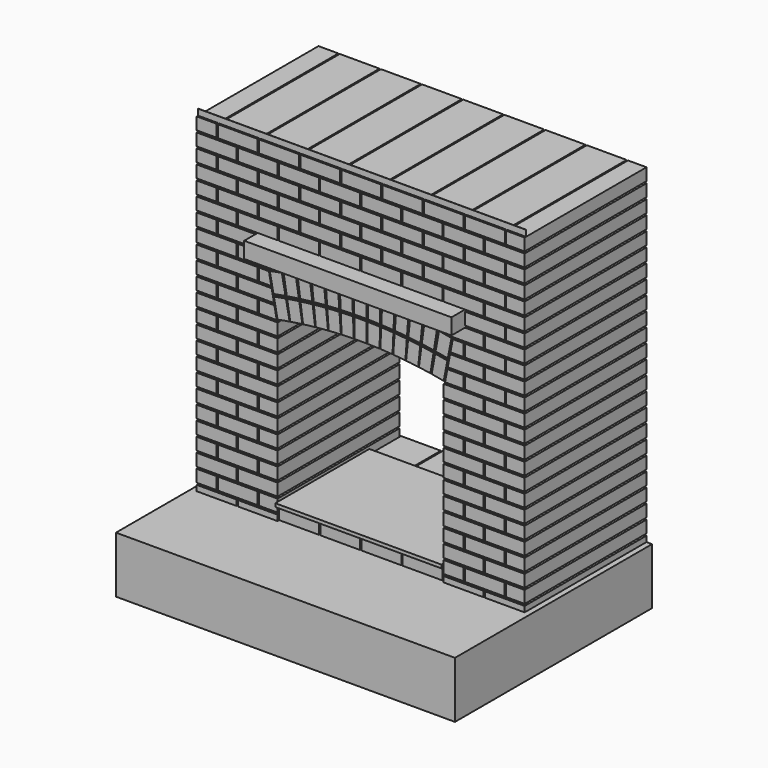
from build123d import *

# Parameters (mm, degrees)
F0_W          = 105.75
F0_H          = 65
F0_W_2        = 211.5
F0_W_3        = 98.25
F0_H_2        = 30
F0_W_4        = 105.25
F0_H_3        = 64.607629
F1_DEPTH      = 10
F1_DEPTH_BACK = 800
F2_DEPTH      = 25
F2_DEPTH_BACK = 600
F3_DEPTH      = 100
F4_DEPTH      = 510
F4_DEPTH_BACK = 800
F5_DEPTH      = 1


# Not quite as in the source:
# - ends of sketch curves that miss each other by under 0.0002 mm in the source are joined


with BuildPart() as f1:
    # F0 (on Front) → F1 (new body, two sides)
    with BuildSketch(Plane.XZ) as f1_sk:
        with Locations((-819.625, 978.6495302)):
            Rectangle(F0_W, F0_H)
        with Locations((-653.5, 978.6495302)):
            Rectangle(F0_W_2, F0_H)
        with Locations((-434.5, 978.6495302)):
            Rectangle(F0_W_2, F0_H)
        with Locations((-215.5, 978.6495302)):
            Rectangle(F0_W_2, F0_H)
        with Locations((3.5, 978.6495302)):
            Rectangle(F0_W_2, F0_H)
        with Locations((222.5, 978.6495302)):
            Rectangle(F0_W_2, F0_H)
        with Locations((441.5, 978.6495302)):
            Rectangle(F0_W_2, F0_H)
        with Locations((660.5, 978.6495302)):
            Rectangle(F0_W_2, F0_H)
        with Locations((822.875, 978.6495302)):
            Rectangle(F0_W_3, F0_H)
        with Locations((766.25, 903.6495302)):
            Rectangle(F0_W_2, F0_H)
        with Locations((-766.75, 903.6495302)):
            Rectangle(F0_W_2, F0_H)
        with Locations((-819.625, 828.6495302)):
            Rectangle(F0_W, F0_H)
        with Locations((-766.75, 753.6495302)):
            Rectangle(F0_W_2, F0_H)
        with Locations((-653.5, 828.6495302)):
            Rectangle(F0_W_2, F0_H)
        with Locations((-547.75, 903.6495302)):
            Rectangle(F0_W_2, F0_H)
        with Locations((-328.75, 903.6495302)):
            Rectangle(F0_W_2, F0_H)
        with Locations((-434.5, 828.6495302)):
            Rectangle(F0_W_2, F0_H)
        with Locations((-547.75, 753.6495302)):
            Rectangle(F0_W_2, F0_H)
        with Locations((-328.75, 753.6495302)):
            Rectangle(F0_W_2, F0_H)
        with Locations((-215.5, 828.6495302)):
            Rectangle(F0_W_2, F0_H)
        with Locations((-109.75, 903.6495302)):
            Rectangle(F0_W_2, F0_H)
        Polygon((-102.25, 861.1495302), (-102.25, 796.1495302), (109.25, 796.1495302), (109.25, 861.1495302), (3.5, 861.1495302), align=None)
        with Locations((-109.75, 753.6495302)):
            Rectangle(F0_W_2, F0_H)
        with Locations((109.25, 903.6495302)):
            Rectangle(F0_W_2, F0_H)
        Polygon((215, 861.1495302), (116.75, 861.1495302), (116.75, 796.1495302), (328.25, 796.1495302), (328.25, 861.1495302), align=None)
        with Locations((328.25, 903.6495302)):
            Rectangle(F0_W_2, F0_H)
        with Locations((441.5, 828.6495302)):
            Rectangle(F0_W_2, F0_H)
        with Locations((328.25, 753.6495302)):
            Rectangle(F0_W_2, F0_H)
        with Locations((547.25, 753.6495302)):
            Rectangle(F0_W_2, F0_H)
        with Locations((822.875, 828.6495302)):
            Rectangle(F0_W_3, F0_H)
        with Locations((766.25, 753.6495302)):
            Rectangle(F0_W_2, F0_H)
        with Locations((547.25, 903.6495302)):
            Rectangle(F0_W_2, F0_H)
        with Locations((660.5, 828.6495302)):
            Rectangle(F0_W_2, F0_H)
        with Locations((109.25, 753.6495302)):
            Rectangle(F0_W_2, F0_H)
        with Locations((-819.625, 678.6495302)):
            Rectangle(F0_W, F0_H)
        with Locations((-766.75, 603.6495302)):
            Rectangle(F0_W_2, F0_H)
        with Locations((-819.625, 528.6495302)):
            Rectangle(F0_W, F0_H)
        with Locations((-653.5, 528.6495302)):
            Rectangle(F0_W_2, F0_H)
        with Locations((-653.5, 678.6495302)):
            Rectangle(F0_W_2, F0_H)
        Polygon((-547.75, 571.1495302), (-442, 571.1495302), (-442, 636.1495302), (-653.5, 636.1495302), (-653.5, 571.1495302), align=None)
        with Locations((-434.5, 678.6495302)):
            Rectangle(F0_W_2, F0_H)
        with Locations((-328.75, 603.6495302)):
            Rectangle(F0_W_2, F0_H)
        with Locations((-215.5, 678.6495302)):
            Rectangle(F0_W_2, F0_H)
        with Locations((-109.75, 603.6495302)):
            Rectangle(F0_W_2, F0_H)
        with Locations((3.5, 678.6495302)):
            Rectangle(F0_W_2, F0_H)
        with Locations((109.25, 603.6495302)):
            Rectangle(F0_W_2, F0_H)
        with Locations((222.5, 678.6495302)):
            Rectangle(F0_W_2, F0_H)
        with Locations((328.25, 603.6495302)):
            Rectangle(F0_W_2, F0_H)
        with Locations((441.5, 678.6495302)):
            Rectangle(F0_W_2, F0_H)
        Polygon((441.5, 636.1495302), (441.5, 571.1495302), (554.75, 571.1495302), (653, 571.1495302), (653, 636.1495302), align=None)
        with Locations((660.5, 678.6495302)):
            Rectangle(F0_W_2, F0_H)
        with Locations((766.25, 603.6495302)):
            Rectangle(F0_W_2, F0_H)
        with Locations((822.875, 678.6495302)):
            Rectangle(F0_W_3, F0_H)
        with Locations((822.875, 528.6495302)):
            Rectangle(F0_W_3, F0_H)
        with Locations((660.5, 528.6495302)):
            Rectangle(F0_W_2, F0_H)
        with Locations((766.25, 453.6495302)):
            Rectangle(F0_W_2, F0_H)
        with BuildLine():
            Line((653, 486.1495302), (554.75, 486.1495302))
            Line((554.75, 486.1495302), (441.5, 486.1495302))
            Line((441.5, 486.1495302), (441.5, 429.1941382))
            ThreePointArc((441.5, 429.1941382), (463.318790633, 425.2664700416), (485.1026609901, 421.1495301488))
            Line((485.1026609901, 421.1495301488), (653, 421.1495302))
            Line((653, 421.1495302), (653, 486.1495302))
        make_face()
        with BuildLine():
            Line((434, 486.1495302), (222.5, 486.1495302))
            Line((222.5, 486.1495302), (222.5, 457.9377232))
            ThreePointArc((222.5, 457.9377232), (328.5365757301, 446.427387097), (434.0000000545, 430.4991305158))
            Line((434.0000000545, 430.4991305158), (434, 486.1495302))
        make_face()
        with BuildLine():
            Line((215, 486.1495302), (3.5, 486.1495302))
            Line((3.5, 486.1495302), (3.5, 467.6471312))
            ThreePointArc((3.5, 467.6471312), (109.3439714945, 465.3074471343), (215.0000000335, 458.582563596))
            Line((215.0000000335, 458.582563596), (215, 486.1495302))
        make_face()
        with BuildLine():
            Line((-4, 486.1495302), (-215.5, 486.1495302))
            Line((-215.5, 486.1495302), (-215.5, 458.5402672))
            ThreePointArc((-215.5, 458.5402672), (-109.8444031396, 465.2859502256), (-4.0000000003, 467.6463973929))
            Line((-4.0000000003, 467.6463973929), (-4, 486.1495302))
        make_face()
        with BuildLine():
            Line((-223, 486.1495302), (-434.5, 486.1495302))
            Line((-434.5, 486.1495302), (-434.5, 430.4128472))
            ThreePointArc((-434.5, 430.4128472), (-329.0370270242, 446.3624116177), (-223.0000000156, 457.8939413783))
            Line((-223.0000000156, 457.8939413783), (-223, 486.1495302))
        make_face()
        with BuildLine():
            Line((-442, 486.1495302), (-547.75, 486.1495302))
            Line((-547.75, 486.1495302), (-653.5, 486.1495302))
            Line((-653.5, 486.1495302), (-653.5, 421.1495302))
            Line((-653.5, 421.1495302), (-485.102661, 421.1495302))
            ThreePointArc((-485.1026609901, 421.1495301488), (-463.5684023211, 425.2204043328), (-442.0000000078, 429.1063192442))
            Line((-442, 429.1063192), (-442, 486.1495302))
        make_face()
        with Locations((-766.75, 453.6495302)):
            Rectangle(F0_W_2, F0_H)
        with Locations((-819.625, 378.6495302)):
            Rectangle(F0_W, F0_H)
        with Locations((-653.5, 378.6495302)):
            Rectangle(F0_W_2, F0_H)
        Polygon((-540.25, 346.1495302), (-475.3907933178, 346.1495302), (-487.9598097393, 411.1495302), (-540.25, 411.1495302), align=None)
        with Locations((-766.75, 303.6495302)):
            Rectangle(F0_W_2, F0_H)
        Polygon((-653.5, 271.1495302), (-460.8880820622, 271.1495302), (-473.4570984837, 336.1495302), (-653.5, 336.1495302), align=None)
        with Locations((-819.625, 228.6495302)):
            Rectangle(F0_W, F0_H)
        with Locations((-653.5, 228.6495302)):
            Rectangle(F0_W_2, F0_H)
        Polygon((-540.25, 196.1495302), (-446.3853708065, 196.1495302), (-446.909066112, 198.8577926219), (-458.9543872281, 261.1495302), (-540.25, 261.1495302), align=None)
        with Locations((-766.75, 153.6495302)):
            Rectangle(F0_W_2, F0_H)
        with Locations((-547.75, 153.6495302)):
            Rectangle(F0_W_2, F0_H)
        with Locations((-819.625, 78.6495302)):
            Rectangle(F0_W, F0_H)
        with Locations((-653.5, 78.6495302)):
            Rectangle(F0_W_2, F0_H)
        with Locations((-491.125, 78.6495302)):
            Rectangle(F0_W_3, F0_H)
        with Locations((-766.75, 3.6495302)):
            Rectangle(F0_W_2, F0_H)
        with Locations((-547.75, 3.6495302)):
            Rectangle(F0_W_2, F0_H)
        with Locations((-819.625, -71.3504698)):
            Rectangle(F0_W, F0_H)
        with Locations((-653.5, -71.3504698)):
            Rectangle(F0_W_2, F0_H)
        with Locations((-491.125, -71.3504698)):
            Rectangle(F0_W_3, F0_H)
        with Locations((-766.75, -146.3504698)):
            Rectangle(F0_W_2, F0_H)
        with Locations((-547.75, -146.3504698)):
            Rectangle(F0_W_2, F0_H)
        with Locations((-819.625, -221.3504698)):
            Rectangle(F0_W, F0_H)
        with Locations((-653.5, -221.3504698)):
            Rectangle(F0_W_2, F0_H)
        with Locations((-491.125, -221.3504698)):
            Rectangle(F0_W_3, F0_H)
        with Locations((-766.75, -296.3504698)):
            Rectangle(F0_W_2, F0_H)
        with Locations((-547.75, -296.3504698)):
            Rectangle(F0_W_2, F0_H)
        with Locations((-819.625, -371.3504698)):
            Rectangle(F0_W, F0_H)
        with Locations((-653.5, -371.3504698)):
            Rectangle(F0_W_2, F0_H)
        with Locations((-491.125, -371.3504698)):
            Rectangle(F0_W_3, F0_H)
        with Locations((-766.75, -446.3504698)):
            Rectangle(F0_W_2, F0_H)
        with Locations((-547.75, -446.3504698)):
            Rectangle(F0_W_2, F0_H)
        with Locations((-819.625, -521.3504698)):
            Rectangle(F0_W, F0_H)
        with Locations((-653.5, -521.3504698)):
            Rectangle(F0_W_2, F0_H)
        with Locations((-491.125, -521.3504698)):
            Rectangle(F0_W_3, F0_H)
        with Locations((-766.75, -596.3504698)):
            Rectangle(F0_W_2, F0_H)
        Polygon((-540.25, -628.8504698), (-442, -628.8504698), (-442, -563.8504698), (-540.25, -563.8504698), (-653.5, -563.8504698), (-653.5, -628.8504698), align=None)
        with Locations((-819.625, -671.3504698)):
            Rectangle(F0_W, F0_H)
        with Locations((-653.5, -671.3504698)):
            Rectangle(F0_W_2, F0_H)
        Polygon((-442, -671.8504698), (-442, -653.8504698), (-442, -638.8504698), (-540.25, -638.8504698), (-540.25, -703.8504698), (-442, -703.8504698), align=None)
        with Locations((-766.75, -728.8504698)):
            Rectangle(F0_W_2, F0_H_2)
        Polygon((-442, -743.8504698), (-442, -713.8504698), (-540.25, -713.8504698), (-653.5, -713.8504698), (-653.5, -743.8504698), align=None)
        with BuildLine():
            Line((-483.387866, 413.8422042), (-463.8330486219, 312.7155060601))
            ThreePointArc((-463.8330486219, 312.7155060601), (-431.8802658345, 318.6739780372), (-399.8510400321, 324.2068283936))
            Line((-399.8510400321, 324.2068283936), (-419.570047, 426.1826232))
            Line((-419.570047, 426.1826232), (-483.387866, 413.8422042))
        make_face()
        with BuildLine():
            ThreePointArc((-442.0000000511, 199.8070564643), (-410.0449024045, 205.7550928325), (-378.0098779423, 211.2564208495))
            Line((-378.0098779423, 211.2564208495), (-397.571998, 312.4208842))
            ThreePointArc((-397.571998, 312.4208842), (-429.6018040146, 306.891183884), (-461.5548179058, 300.933754713))
            Line((-461.5548179058, 300.933754713), (-442.0000000511, 199.8070564643))
        make_face()
        with BuildLine():
            Line((-345.255049, 436.6325702), (-409.542155, 426.9963582))
            Line((-409.542155, 426.9963582), (-392.97466, 325.3375522))
            ThreePointArc((-392.97466, 325.3375522), (-360.8602260561, 330.3522189595), (-328.6819200208, 334.9391973533))
            Line((-328.6819200208, 334.9391973533), (-345.255049, 436.6325702))
        make_face()
        with BuildLine():
            ThreePointArc((-374.4769660256, 211.8349733574), (-342.3605263553, 216.8391409049), (-310.1773530512, 221.3944395805))
            Line((-310.1773530512, 221.3944395805), (-326.751039, 323.0912352))
            ThreePointArc((-326.751039, 323.0912352), (-358.9298321954, 318.5074223666), (-391.044466044, 313.4938044698))
            Line((-391.044466044, 313.4938044698), (-374.4769660256, 211.8349733574))
        make_face()
        with BuildLine():
            ThreePointArc((-321.7752320422, 335.8668735179), (-289.5270191307, 339.933383771), (-257.2275600242, 343.5705094282))
            Line((-257.2275600242, 343.5705094282), (-270.797958, 445.7079412))
            Line((-270.797958, 445.7079412), (-335.341018, 437.9695962))
            Line((-335.341018, 437.9695962), (-321.7752320422, 335.8668735179))
        make_face()
        with BuildLine():
            ThreePointArc((-306.6289640133, 221.8686693005), (-274.3790547682, 225.9246255739), (-242.0756629788, 229.5299419976))
            Line((-242.0756629788, 229.5299419976), (-255.646518, 331.6708112))
            ThreePointArc((-255.646518, 331.6708112), (-287.9463704388, 328.0368642661), (-320.1947519369, 323.9714087251))
            Line((-320.1947519369, 323.9714087251), (-306.6289640133, 221.8686693005))
        make_face()
        with BuildLine():
            Line((-196.016445, 452.5930292), (-260.759648, 446.7615452))
            Line((-260.759648, 446.7615452), (-250.210954, 344.3031492))
            ThreePointArc((-250.210954, 344.3031492), (-217.8568398047, 347.4168338833), (-185.4641650184, 350.0998094411))
            Line((-185.4641650184, 350.0998094411), (-196.016445, 452.5930292))
        make_face()
        with BuildLine():
            ThreePointArc((-238.433284987, 229.9078410742), (-206.0777865672, 233.0109264045), (-173.6821190309, 235.661990613))
            Line((-173.6821190309, 235.661990613), (-184.234754, 338.1586602))
            ThreePointArc((-184.234754, 338.1586602), (-216.6277282892, 335.4788729431), (-248.9819800237, 332.3662474302))
            Line((-248.9819800237, 332.3662474302), (-238.433284987, 229.9078410742))
        make_face()
        with BuildLine():
            Line((-121.064406, 457.2696832), (-185.951429, 453.3501322))
            Line((-185.951429, 453.3501322), (-178.429004, 350.6251982))
            ThreePointArc((-178.429004, 350.6251982), (-145.9971352331, 352.7833488419), (-113.5394250016, 354.5098402354))
            Line((-113.5394250016, 354.5098402354), (-121.064406, 457.2696832))
        make_face()
        with BuildLine():
            ThreePointArc((-170.0301799999, 235.9323051992), (-137.5972403613, 238.0798200442), (-105.1374799791, 239.7743257379))
            Line((-105.1374799791, 239.7743257379), (-112.662714, 342.5376272))
            ThreePointArc((-112.662714, 342.5376272), (-145.120629789, 340.8143319749), (-177.5526050104, 338.6572443423))
            Line((-177.5526050104, 338.6572443423), (-170.0301799999, 235.9323051992))
        make_face()
        with BuildLine():
            Line((-46.007048, 459.7338352), (-110.981441, 457.7296252))
            Line((-110.981441, 457.7296252), (-106.49183, 354.8275212))
            ThreePointArc((-106.49183, 354.8275212), (-74.0104204152, 356.0282600205), (-41.5159110018, 356.7967653066))
            Line((-41.5159110018, 356.7967653066), (-46.007048, 459.7338352))
        make_face()
        with BuildLine():
            ThreePointArc((-75.0000000044, 240.9411613357), (-55.7525948236, 241.4818680956), (-36.5013759947, 241.8633698602))
            Line((-36.5013759947, 241.8633698602), (-40.992664, 344.8039042))
            ThreePointArc((-40.992664, 344.8039042), (-73.4872844958, 344.0385996794), (-105.9687690118, 342.8389264701))
            Line((-105.9687690118, 342.8389264701), (-101.479157, 239.9368202))
            ThreePointArc((-101.479157, 239.9368202), (-88.2410074228, 240.4766638217), (-75.0000000044, 240.9411613357))
        make_face()
        with BuildLine():
            Line((29.090335, 459.9833412), (-35.914904, 459.8962142))
            Line((-35.914904, 459.8962142), (-34.462013, 356.9064622))
            ThreePointArc((-34.4620130003, 356.9064622227), (-1.9593204, 357.1487445378), (30.5437189994, 356.9585951494))
            Line((30.543719, 356.9585952), (29.090335, 459.9833412))
        make_face()
        with BuildLine():
            ThreePointArc((-32.8398530067, 241.9179036746), (-0.3367183175, 242.1495058501), (32.1664820055, 241.9273055979))
            Line((32.1664820055, 241.9273055979), (30.713049, 344.9555192))
            ThreePointArc((30.713049, 344.9555192), (-1.7900074832, 345.1488712188), (-34.2927439988, 344.9076561152))
            Line((-34.2927439988, 344.9076561152), (-32.8398530067, 241.9179036746))
        make_face()
        with BuildLine():
            Line((104.16241, 458.0179842), (39.182878, 459.8480152))
            Line((39.182878, 459.8480152), (37.597785, 356.8602122))
            ThreePointArc((37.597785, 356.8602122), (70.0934852596, 356.143827617), (102.5767789897, 354.9951889544))
            Line((102.5767789897, 354.9951889544), (104.16241, 458.0179842))
        make_face()
        with BuildLine():
            ThreePointArc((75.0000000044, 240.9411613357), (87.9045305346, 240.4894018482), (100.8063570059, 239.9660773369))
            Line((100.8063570059, 239.9660773369), (102.392042, 342.9923402))
            ThreePointArc((102.392042, 342.9923402), (69.9088261653, 344.1441806532), (37.4131140046, 344.8616334979))
            Line((37.4131140046, 344.8616334979), (35.828021, 241.8738312))
            ThreePointArc((35.828021, 241.8738312), (55.4159726779, 241.4899072947), (75.0000000044, 240.9411613357))
        make_face()
        with BuildLine():
            Line((179.143869, 453.8394742), (114.246572, 457.5850682))
            Line((114.246572, 457.5850682), (109.624874, 354.6888122))
            ThreePointArc((109.624874, 354.6888122), (142.0853120166, 353.0143835036), (174.520600974, 350.9082548371))
            Line((174.520600974, 350.9082548371), (179.143869, 453.8394742))
        make_face()
        with BuildLine():
            ThreePointArc((104.4647260219, 239.8046406883), (136.9249753655, 238.1195244227), (169.3585350045, 235.981391262))
            Line((169.3585350045, 235.981391262), (173.981959, 338.9160752))
            ThreePointArc((173.981959, 338.9160752), (141.5468423868, 341.0254020347), (109.0864240213, 342.7008986747))
            Line((109.0864240213, 342.7008986747), (104.4647260219, 239.8046406883))
        make_face()
        with BuildLine():
            Line((253.969481, 447.4514462), (189.210877, 453.1093432))
            Line((189.210877, 453.1093432), (181.556595, 350.3941502))
            ThreePointArc((181.556595, 350.3941502), (213.9535313724, 347.763134652), (246.3125980045, 344.7013482448))
            Line((246.3125980045, 344.7013482448), (253.969481, 447.4514462))
        make_face()
        with BuildLine():
            ThreePointArc((173.0105519895, 235.7121330592), (205.4069846582, 233.0704398176), (237.7633789655, 229.976713864))
            Line((237.7633789655, 229.976713864), (245.42052, 332.7302702))
            ThreePointArc((245.42052, 332.7302702), (213.0617195995, 335.7952485431), (180.6648340136, 338.427331383))
            Line((180.6648340136, 338.427331383), (173.0105519895, 235.7121330592))
        make_face()
        with BuildLine():
            Line((328.574151, 438.8594582), (264.010577, 446.4247342))
            Line((264.010577, 446.4247342), (253.33037, 343.9799632))
            ThreePointArc((253.33037, 343.9799632), (285.6356212129, 340.3946494003), (317.8903149526, 336.3798688386))
            Line((317.8903149526, 336.3798688386), (328.574151, 438.8594582))
        make_face()
        with BuildLine():
            Line((305.961381, 221.9572692), (316.645576, 324.4403072))
            ThreePointArc((316.645576, 324.4403072), (284.3912427335, 328.4582702099), (252.0860740238, 332.0446494287))
            Line((252.0860740238, 332.0446494287), (241.405867, 229.5998682))
            ThreePointArc((241.405867, 229.5998682), (273.7103000729, 226.0038961985), (305.961381, 221.9572692))
        make_face()
        with BuildLine():
            Line((405.599474, 427.6357542), (338.580599, 437.5370562))
            Line((338.580599, 437.5370562), (324.88376, 335.4518312))
            ThreePointArc((324.88376, 335.4518312), (357.0692220657, 330.9153378912), (389.1914829385, 325.9510558191))
            Line((389.1914829385, 325.9510558191), (405.599474, 427.6357542))
        make_face()
        with BuildLine():
            Line((323.288012, 323.5584052), (309.59117, 221.4731632))
            ThreePointArc((309.59117, 221.4731632), (340.2616386282, 217.1502064186), (370.8718809386, 212.4195968195))
            Line((370.8718809386, 212.4195968195), (387.279872, 314.1042952))
            ThreePointArc((387.279872, 314.1042952), (355.3153873438, 319.044193727), (323.288012, 323.5584052))
        make_face()
        with BuildLine():
            ThreePointArc((398.2221910504, 324.4764905053), (430.8047181498, 318.8669007094), (463.3083509699, 312.8169070443))
            Line((463.3083509699, 312.8169070443), (482.841047, 413.9478802))
            Line((482.841047, 413.9478802), (416.775209, 425.8069112))
            Line((416.775209, 425.8069112), (398.2221910504, 324.4764905053))
        make_face()
        with BuildLine():
            Line((396.060659, 312.6709242), (377.507375, 211.3390512))
            ThreePointArc((377.507375, 211.3390512), (409.5436020977, 205.8447308744), (441.5000000537, 199.9036844779))
            Line((441.5000000537, 199.9036844779), (461.0326965703, 301.0346578085))
            ThreePointArc((461.0326965703, 301.0346578085), (428.5861708433, 307.0733027072), (396.060659, 312.6709242))
        make_face()
        Polygon((477.384909, 346.1495302), (547.25, 346.1495302), (547.25, 411.1495302), (489.939176, 411.1495302), align=None)
        with Locations((660.5, 378.6495302)):
            Rectangle(F0_W_2, F0_H)
        with Locations((822.875, 378.6495302)):
            Rectangle(F0_W_3, F0_H)
        Polygon((462.899216, 271.1495302), (653, 271.1495302), (653, 336.1495302), (475.453483, 336.1495302), align=None)
        with Locations((766.25, 303.6495302)):
            Rectangle(F0_W_2, F0_H)
        Polygon((448.413522, 196.1495302), (547.25, 196.1495302), (547.25, 261.1495302), (460.96779, 261.1495302), align=None)
        with Locations((660.5, 228.6495302)):
            Rectangle(F0_W_2, F0_H)
        with Locations((822.875, 228.6495302)):
            Rectangle(F0_W_3, F0_H)
        with Locations((547.25, 153.6495302)):
            Rectangle(F0_W_2, F0_H)
        with Locations((766.25, 153.6495302)):
            Rectangle(F0_W_2, F0_H)
        with Locations((494.125, 78.6495302)):
            Rectangle(F0_W_4, F0_H)
        Polygon((554.25, 46.1495302), (765.75, 46.1495302), (765.75, 111.1495302), (660.5, 111.1495302), (554.25, 111.1495302), align=None)
        Polygon((871.5, 46.1495302), (872, 46.1495302), (872, 111.1495302), (773.25, 111.1495302), (773.25, 46.1495302), align=None)
        with Locations((547.25, 3.6495302)):
            Rectangle(F0_W_2, F0_H)
        with Locations((766.25, 3.6495302)):
            Rectangle(F0_W_2, F0_H)
        with Locations((494.125, -71.3504698)):
            Rectangle(F0_W_4, F0_H)
        Polygon((554.25, -103.8504698), (765.75, -103.8504698), (765.75, -38.8504698), (660.5, -38.8504698), (554.25, -38.8504698), align=None)
        Polygon((871.5, -103.8504698), (872, -103.8504698), (872, -38.8504698), (773.25, -38.8504698), (773.25, -103.8504698), align=None)
        with Locations((547.25, -146.3504698)):
            Rectangle(F0_W_2, F0_H)
        with Locations((766.25, -146.3504698)):
            Rectangle(F0_W_2, F0_H)
        with Locations((494.125, -221.3504698)):
            Rectangle(F0_W_4, F0_H)
        Polygon((554.25, -253.8504698), (765.75, -253.8504698), (765.75, -188.8504698), (660.5, -188.8504698), (554.25, -188.8504698), align=None)
        Polygon((871.5, -253.8504698), (872, -253.8504698), (872, -188.8504698), (773.25, -188.8504698), (773.25, -253.8504698), align=None)
        with Locations((547.25, -296.3504698)):
            Rectangle(F0_W_2, F0_H)
        with Locations((766.25, -296.3504698)):
            Rectangle(F0_W_2, F0_H)
        with Locations((494.125, -371.3504698)):
            Rectangle(F0_W_4, F0_H)
        Polygon((554.25, -403.8504698), (765.75, -403.8504698), (765.75, -338.8504698), (660.5, -338.8504698), (554.25, -338.8504698), align=None)
        Polygon((871.5, -403.8504698), (872, -403.8504698), (872, -338.8504698), (773.25, -338.8504698), (773.25, -403.8504698), align=None)
        with Locations((547.25, -446.3504698)):
            Rectangle(F0_W_2, F0_H)
        with Locations((766.25, -446.3504698)):
            Rectangle(F0_W_2, F0_H)
        with Locations((494.125, -521.3504698)):
            Rectangle(F0_W_4, F0_H)
        Polygon((554.25, -553.8504698), (765.75, -553.8504698), (765.75, -488.8504698), (660.5, -488.8504698), (554.25, -488.8504698), align=None)
        Polygon((871.5, -553.8504698), (872, -553.8504698), (872, -488.8504698), (773.25, -488.8504698), (773.25, -553.8504698), align=None)
        with Locations((547.25, -596.3504698)):
            Rectangle(F0_W_2, F0_H)
        with Locations((766.25, -596.3504698)):
            Rectangle(F0_W_2, F0_H)
        Polygon((546.75, -638.8504698), (441.5, -638.8504698), (441.5, -653.8504698), (441.5, -671.8504698), (441.5, -703.8504698), (546.75, -703.8504698), align=None)
        Polygon((554.25, -703.8504698), (765.75, -703.8504698), (765.75, -638.8504698), (660.5, -638.8504698), (554.25, -638.8504698), align=None)
        Polygon((871.5, -703.8504698), (872, -703.8504698), (872, -638.8504698), (773.25, -638.8504698), (773.25, -703.8504698), align=None)
        with Locations((547.25, -728.8504698)):
            Rectangle(F0_W_2, F0_H_2)
        with Locations((766.25, -728.8504698)):
            Rectangle(F0_W_2, F0_H_2)
        with Locations((-327.566109, -704.1542843)):
            Rectangle(F0_W_2, F0_H_3)
        Polygon((-2.816109, -671.8504698), (-214.316109, -671.8504698), (-214.316109, -736.4580988), (-101.066109, -736.4580988), (-2.816109, -736.4580988), align=None)
        with Locations((110.433891, -704.1542843)):
            Rectangle(F0_W_2, F0_H_3)
        with Locations((329.433891, -704.1542843)):
            Rectangle(F0_W_2, F0_H_3)
    extrude(amount=F1_DEPTH)
    extrude(f1_sk.sketch, amount=-F1_DEPTH_BACK)


with BuildPart() as f2:
    # F0 (on Front) → F2 (new body, two sides)
    with BuildSketch(Plane.XZ) as f2_sk:
        Polygon((441.5, -671.8504698), (441.5, -653.8504698), (-442, -653.8504698), (-442, -671.8504698), (-433.316109, -671.8504698), (-221.816109, -671.8504698), (-214.316109, -671.8504698), (-2.816109, -671.8504698), (4.683891, -671.8504698), (216.183891, -671.8504698), (223.683891, -671.8504698), (435.183891, -671.8504698), align=None)
    extrude(amount=F2_DEPTH)
    extrude(f2_sk.sketch, amount=-F2_DEPTH_BACK)


with BuildPart() as f3:
    # F0 (on Front) → F3 (new body)
    with BuildSketch(Plane.XZ):
        Polygon((-434.5, 571.1495302), (-442, 571.1495302), (-547.75, 571.1495302), (-547.75, 561.1495302), (-547.75, 496.1495302), (-547.75, 486.1495302), (-442, 486.1495302), (-434.5, 486.1495302), (-223, 486.1495302), (-215.5, 486.1495302), (-4, 486.1495302), (3.5, 486.1495302), (215, 486.1495302), (222.5, 486.1495302), (434, 486.1495302), (441.5, 486.1495302), (554.75, 486.1495302), (554.75, 496.1495302), (554.75, 561.1495302), (554.75, 571.1495302), (441.5, 571.1495302), (434, 571.1495302), (222.5, 571.1495302), (215, 571.1495302), (3.5, 571.1495302), (-4, 571.1495302), (-215.5, 571.1495302), (-223, 571.1495302), align=None)
    extrude(amount=F3_DEPTH)


with BuildPart() as f4:
    # F0 (on Front) → F4 (new body, two sides)
    with BuildSketch(Plane.XZ) as f4_sk:
        Polygon((653, -743.8504698), (441.5, -743.8504698), (2.5, -743.8504698), (-95.75, -743.8504698), (-103.25, -743.8504698), (-314.75, -743.8504698), (-322.25, -743.8504698), (-428, -743.8504698), (-442, -743.8504698), (-653.5, -743.8504698), (-661, -743.8504698), (-872.5, -743.8504698), (-901.5, -743.8504698), (-901.5, -1043.8504698), (901.5, -1043.8504698), (901.5, -743.8504698), (872, -743.8504698), (660.5, -743.8504698), align=None)
    extrude(amount=F4_DEPTH)
    extrude(f4_sk.sketch, amount=-F4_DEPTH_BACK)


with BuildPart() as f5:
    # F0 (on Front) → F5 (new body)
    with BuildSketch(Plane.XZ):
        with BuildLine():
            ThreePointArc((252.0860740238, 332.0446494287), (284.3912427335, 328.4582702099), (316.6455760142, 324.4403073079))
            Line((316.6455760142, 324.4403073079), (305.961381, 221.9572692))
            ThreePointArc((305.961381, 221.9572692), (307.7763706985, 221.7159299891), (309.5911700875, 221.4731638524))
            Line((309.5911700875, 221.4731638524), (323.288012, 323.5584052))
            ThreePointArc((323.288012, 323.5584052), (355.3153873438, 319.044193727), (387.2798719572, 314.1042949345))
            Line((387.2798719572, 314.1042949345), (370.871881, 212.4195972))
            ThreePointArc((370.871881, 212.4195972), (374.190018025, 211.8817192921), (377.5073750406, 211.3390514471))
            Line((377.5073750406, 211.3390514471), (396.060659, 312.6709242))
            ThreePointArc((396.060659, 312.6709242), (428.5861708433, 307.0733027072), (461.0326969117, 301.0346577426))
            Line((461.0326969117, 301.0346577426), (441.5, 199.9036842))
            Line((441.5, 199.9036842), (441.5, 186.1495302))
            Line((441.5, 186.1495302), (653, 186.1495302))
            Line((653, 186.1495302), (653, 121.1495302))
            Line((653, 121.1495302), (441.5, 121.1495302))
            Line((441.5, 121.1495302), (441.5, 111.1495302))
            Line((441.5, 111.1495302), (546.75, 111.1495302))
            Line((546.75, 111.1495302), (546.75, 46.1495302))
            Line((546.75, 46.1495302), (441.5, 46.1495302))
            Line((441.5, 46.1495302), (441.5, 36.1495302))
            Line((441.5, 36.1495302), (653, 36.1495302))
            Line((653, 36.1495302), (653, -28.8504698))
            Line((653, -28.8504698), (441.5, -28.8504698))
            Line((441.5, -28.8504698), (441.5, -38.8504698))
            Line((441.5, -38.8504698), (546.75, -38.8504698))
            Line((546.75, -38.8504698), (546.75, -103.8504698))
            Line((546.75, -103.8504698), (441.5, -103.8504698))
            Line((441.5, -103.8504698), (441.5, -113.8504698))
            Line((441.5, -113.8504698), (653, -113.8504698))
            Line((653, -113.8504698), (653, -178.8504698))
            Line((653, -178.8504698), (441.5, -178.8504698))
            Line((441.5, -178.8504698), (441.5, -188.8504698))
            Line((441.5, -188.8504698), (546.75, -188.8504698))
            Line((546.75, -188.8504698), (546.75, -253.8504698))
            Line((546.75, -253.8504698), (441.5, -253.8504698))
            Line((441.5, -253.8504698), (441.5, -263.8504698))
            Line((441.5, -263.8504698), (653, -263.8504698))
            Line((653, -263.8504698), (653, -328.8504698))
            Line((653, -328.8504698), (441.5, -328.8504698))
            Line((441.5, -328.8504698), (441.5, -338.8504698))
            Line((441.5, -338.8504698), (546.75, -338.8504698))
            Line((546.75, -338.8504698), (546.75, -403.8504698))
            Line((546.75, -403.8504698), (441.5, -403.8504698))
            Line((441.5, -403.8504698), (441.5, -413.8504698))
            Line((441.5, -413.8504698), (653, -413.8504698))
            Line((653, -413.8504698), (653, -478.8504698))
            Line((653, -478.8504698), (441.5, -478.8504698))
            Line((441.5, -478.8504698), (441.5, -488.8504698))
            Line((441.5, -488.8504698), (546.75, -488.8504698))
            Line((546.75, -488.8504698), (546.75, -553.8504698))
            Line((546.75, -553.8504698), (441.5, -553.8504698))
            Line((441.5, -553.8504698), (441.5, -563.8504698))
            Line((441.5, -563.8504698), (653, -563.8504698))
            Line((653, -563.8504698), (653, -628.8504698))
            Line((653, -628.8504698), (441.5, -628.8504698))
            Line((441.5, -628.8504698), (441.5, -638.8504698))
            Line((441.5, -638.8504698), (546.75, -638.8504698))
            Line((546.75, -638.8504698), (546.75, -703.8504698))
            Line((546.75, -703.8504698), (441.5, -703.8504698))
            Line((441.5, -703.8504698), (441.5, -713.8504698))
            Line((441.5, -713.8504698), (653, -713.8504698))
            Line((653, -713.8504698), (653, -743.8504698))
            Line((653, -743.8504698), (660.5, -743.8504698))
            Line((660.5, -743.8504698), (660.5, -713.8504698))
            Line((660.5, -713.8504698), (872, -713.8504698))
            Line((872, -713.8504698), (872, -703.8504698))
            Line((872, -703.8504698), (871.5, -703.8504698))
            Line((871.5, -703.8504698), (773.25, -703.8504698))
            Line((773.25, -703.8504698), (773.25, -638.8504698))
            Line((773.25, -638.8504698), (872, -638.8504698))
            Line((872, -638.8504698), (872, -628.8504698))
            Line((872, -628.8504698), (660.5, -628.8504698))
            Line((660.5, -628.8504698), (660.5, -563.8504698))
            Line((660.5, -563.8504698), (872, -563.8504698))
            Line((872, -563.8504698), (872, -553.8504698))
            Line((872, -553.8504698), (871.5, -553.8504698))
            Line((871.5, -553.8504698), (773.25, -553.8504698))
            Line((773.25, -553.8504698), (773.25, -488.8504698))
            Line((773.25, -488.8504698), (872, -488.8504698))
            Line((872, -488.8504698), (872, -478.8504698))
            Line((872, -478.8504698), (660.5, -478.8504698))
            Line((660.5, -478.8504698), (660.5, -413.8504698))
            Line((660.5, -413.8504698), (872, -413.8504698))
            Line((872, -413.8504698), (872, -403.8504698))
            Line((872, -403.8504698), (871.5, -403.8504698))
            Line((871.5, -403.8504698), (773.25, -403.8504698))
            Line((773.25, -403.8504698), (773.25, -338.8504698))
            Line((773.25, -338.8504698), (872, -338.8504698))
            Line((872, -338.8504698), (872, -328.8504698))
            Line((872, -328.8504698), (660.5, -328.8504698))
            Line((660.5, -328.8504698), (660.5, -263.8504698))
            Line((660.5, -263.8504698), (872, -263.8504698))
            Line((872, -263.8504698), (872, -253.8504698))
            Line((872, -253.8504698), (871.5, -253.8504698))
            Line((871.5, -253.8504698), (773.25, -253.8504698))
            Line((773.25, -253.8504698), (773.25, -188.8504698))
            Line((773.25, -188.8504698), (872, -188.8504698))
            Line((872, -188.8504698), (872, -178.8504698))
            Line((872, -178.8504698), (660.5, -178.8504698))
            Line((660.5, -178.8504698), (660.5, -113.8504698))
            Line((660.5, -113.8504698), (872, -113.8504698))
            Line((872, -113.8504698), (872, -103.8504698))
            Line((872, -103.8504698), (871.5, -103.8504698))
            Line((871.5, -103.8504698), (773.25, -103.8504698))
            Line((773.25, -103.8504698), (773.25, -38.8504698))
            Line((773.25, -38.8504698), (872, -38.8504698))
            Line((872, -38.8504698), (872, -28.8504698))
            Line((872, -28.8504698), (660.5, -28.8504698))
            Line((660.5, -28.8504698), (660.5, 36.1495302))
            Line((660.5, 36.1495302), (872, 36.1495302))
            Line((872, 36.1495302), (872, 46.1495302))
            Line((872, 46.1495302), (871.5, 46.1495302))
            Line((871.5, 46.1495302), (773.25, 46.1495302))
            Line((773.25, 46.1495302), (773.25, 111.1495302))
            Line((773.25, 111.1495302), (872, 111.1495302))
            Line((872, 111.1495302), (872, 121.1495302))
            Line((872, 121.1495302), (660.5, 121.1495302))
            Line((660.5, 121.1495302), (660.5, 186.1495302))
            Line((660.5, 186.1495302), (872, 186.1495302))
            Line((872, 186.1495302), (872, 196.1495302))
            Line((872, 196.1495302), (773.75, 196.1495302))
            Line((773.75, 196.1495302), (773.75, 261.1495302))
            Line((773.75, 261.1495302), (872, 261.1495302))
            Line((872, 261.1495302), (872, 271.1495302))
            Line((872, 271.1495302), (660.5, 271.1495302))
            Line((660.5, 271.1495302), (660.5, 336.1495302))
            Line((660.5, 336.1495302), (872, 336.1495302))
            Line((872, 336.1495302), (872, 346.1495302))
            Line((872, 346.1495302), (773.75, 346.1495302))
            Line((773.75, 346.1495302), (773.75, 411.1495302))
            Line((773.75, 411.1495302), (872, 411.1495302))
            Line((872, 411.1495302), (872, 421.1495302))
            Line((872, 421.1495302), (660.5, 421.1495302))
            Line((660.5, 421.1495302), (660.5, 486.1495302))
            Line((660.5, 486.1495302), (872, 486.1495302))
            Line((872, 486.1495302), (872, 496.1495302))
            Line((872, 496.1495302), (773.75, 496.1495302))
            Line((773.75, 496.1495302), (773.75, 561.1495302))
            Line((773.75, 561.1495302), (872, 561.1495302))
            Line((872, 561.1495302), (872, 571.1495302))
            Line((872, 571.1495302), (660.5, 571.1495302))
            Line((660.5, 571.1495302), (660.5, 636.1495302))
            Line((660.5, 636.1495302), (872, 636.1495302))
            Line((872, 636.1495302), (872, 646.1495302))
            Line((872, 646.1495302), (773.75, 646.1495302))
            Line((773.75, 646.1495302), (773.75, 711.1495302))
            Line((773.75, 711.1495302), (872, 711.1495302))
            Line((872, 711.1495302), (872, 721.1495302))
            Line((872, 721.1495302), (660.5, 721.1495302))
            Line((660.5, 721.1495302), (660.5, 786.1495302))
            Line((660.5, 786.1495302), (872, 786.1495302))
            Line((872, 786.1495302), (872, 796.1495302))
            Line((872, 796.1495302), (773.75, 796.1495302))
            Line((773.75, 796.1495302), (773.75, 861.1495302))
            Line((773.75, 861.1495302), (872, 861.1495302))
            Line((872, 861.1495302), (872, 871.1495302))
            Line((872, 871.1495302), (660.5, 871.1495302))
            Line((660.5, 871.1495302), (660.5, 936.1495302))
            Line((660.5, 936.1495302), (872, 936.1495302))
            Line((872, 936.1495302), (872, 946.1495302))
            Line((872, 946.1495302), (773.75, 946.1495302))
            Line((773.75, 946.1495302), (773.75, 1011.1495302))
            Line((773.75, 1011.1495302), (872, 1011.1495302))
            Line((872, 1011.1495302), (872, 1043.8504952))
            Line((872, 1043.8504952), (-872.5, 1043.8504952))
            Line((-872.5, 1043.8504952), (-872.5, 1011.1495302))
            Line((-872.5, 1011.1495302), (-766.75, 1011.1495302))
            Line((-766.75, 1011.1495302), (-766.75, 946.1495302))
            Line((-766.75, 946.1495302), (-872.5, 946.1495302))
            Line((-872.5, 946.1495302), (-872.5, 936.1495302))
            Line((-872.5, 936.1495302), (-661, 936.1495302))
            Line((-661, 936.1495302), (-661, 871.1495302))
            Line((-661, 871.1495302), (-872.5, 871.1495302))
            Line((-872.5, 871.1495302), (-872.5, 861.1495302))
            Line((-872.5, 861.1495302), (-766.75, 861.1495302))
            Line((-766.75, 861.1495302), (-766.75, 796.1495302))
            Line((-766.75, 796.1495302), (-872.5, 796.1495302))
            Line((-872.5, 796.1495302), (-872.5, 786.1495302))
            Line((-872.5, 786.1495302), (-661, 786.1495302))
            Line((-661, 786.1495302), (-661, 721.1495302))
            Line((-661, 721.1495302), (-872.5, 721.1495302))
            Line((-872.5, 721.1495302), (-872.5, 711.1495302))
            Line((-872.5, 711.1495302), (-766.75, 711.1495302))
            Line((-766.75, 711.1495302), (-766.75, 646.1495302))
            Line((-766.75, 646.1495302), (-872.5, 646.1495302))
            Line((-872.5, 646.1495302), (-872.5, 636.1495302))
            Line((-872.5, 636.1495302), (-661, 636.1495302))
            Line((-661, 636.1495302), (-661, 571.1495302))
            Line((-661, 571.1495302), (-872.5, 571.1495302))
            Line((-872.5, 571.1495302), (-872.5, 561.1495302))
            Line((-872.5, 561.1495302), (-766.75, 561.1495302))
            Line((-766.75, 561.1495302), (-766.75, 496.1495302))
            Line((-766.75, 496.1495302), (-872.5, 496.1495302))
            Line((-872.5, 496.1495302), (-872.5, 486.1495302))
            Line((-872.5, 486.1495302), (-661, 486.1495302))
            Line((-661, 486.1495302), (-661, 421.1495302))
            Line((-661, 421.1495302), (-872.5, 421.1495302))
            Line((-872.5, 421.1495302), (-872.5, 411.1495302))
            Line((-872.5, 411.1495302), (-766.75, 411.1495302))
            Line((-766.75, 411.1495302), (-766.75, 346.1495302))
            Line((-766.75, 346.1495302), (-872.5, 346.1495302))
            Line((-872.5, 346.1495302), (-872.5, 336.1495302))
            Line((-872.5, 336.1495302), (-661, 336.1495302))
            Line((-661, 336.1495302), (-661, 271.1495302))
            Line((-661, 271.1495302), (-872.5, 271.1495302))
            Line((-872.5, 271.1495302), (-872.5, 261.1495302))
            Line((-872.5, 261.1495302), (-766.75, 261.1495302))
            Line((-766.75, 261.1495302), (-766.75, 196.1495302))
            Line((-766.75, 196.1495302), (-872.5, 196.1495302))
            Line((-872.5, 196.1495302), (-872.5, 186.1495302))
            Line((-872.5, 186.1495302), (-661, 186.1495302))
            Line((-661, 186.1495302), (-661, 121.1495302))
            Line((-661, 121.1495302), (-872.5, 121.1495302))
            Line((-872.5, 121.1495302), (-872.5, 111.1495302))
            Line((-872.5, 111.1495302), (-766.75, 111.1495302))
            Line((-766.75, 111.1495302), (-766.75, 46.1495302))
            Line((-766.75, 46.1495302), (-872.5, 46.1495302))
            Line((-872.5, 46.1495302), (-872.5, 36.1495302))
            Line((-872.5, 36.1495302), (-661, 36.1495302))
            Line((-661, 36.1495302), (-661, -28.8504698))
            Line((-661, -28.8504698), (-872.5, -28.8504698))
            Line((-872.5, -28.8504698), (-872.5, -38.8504698))
            Line((-872.5, -38.8504698), (-766.75, -38.8504698))
            Line((-766.75, -38.8504698), (-766.75, -103.8504698))
            Line((-766.75, -103.8504698), (-872.5, -103.8504698))
            Line((-872.5, -103.8504698), (-872.5, -113.8504698))
            Line((-872.5, -113.8504698), (-661, -113.8504698))
            Line((-661, -113.8504698), (-661, -178.8504698))
            Line((-661, -178.8504698), (-872.5, -178.8504698))
            Line((-872.5, -178.8504698), (-872.5, -188.8504698))
            Line((-872.5, -188.8504698), (-766.75, -188.8504698))
            Line((-766.75, -188.8504698), (-766.75, -253.8504698))
            Line((-766.75, -253.8504698), (-872.5, -253.8504698))
            Line((-872.5, -253.8504698), (-872.5, -263.8504698))
            Line((-872.5, -263.8504698), (-661, -263.8504698))
            Line((-661, -263.8504698), (-661, -328.8504698))
            Line((-661, -328.8504698), (-872.5, -328.8504698))
            Line((-872.5, -328.8504698), (-872.5, -338.8504698))
            Line((-872.5, -338.8504698), (-766.75, -338.8504698))
            Line((-766.75, -338.8504698), (-766.75, -403.8504698))
            Line((-766.75, -403.8504698), (-872.5, -403.8504698))
            Line((-872.5, -403.8504698), (-872.5, -413.8504698))
            Line((-872.5, -413.8504698), (-661, -413.8504698))
            Line((-661, -413.8504698), (-661, -478.8504698))
            Line((-661, -478.8504698), (-872.5, -478.8504698))
            Line((-872.5, -478.8504698), (-872.5, -488.8504698))
            Line((-872.5, -488.8504698), (-766.75, -488.8504698))
            Line((-766.75, -488.8504698), (-766.75, -553.8504698))
            Line((-766.75, -553.8504698), (-872.5, -553.8504698))
            Line((-872.5, -553.8504698), (-872.5, -563.8504698))
            Line((-872.5, -563.8504698), (-661, -563.8504698))
            Line((-661, -563.8504698), (-661, -628.8504698))
            Line((-661, -628.8504698), (-872.5, -628.8504698))
            Line((-872.5, -628.8504698), (-872.5, -638.8504698))
            Line((-872.5, -638.8504698), (-766.75, -638.8504698))
            Line((-766.75, -638.8504698), (-766.75, -703.8504698))
            Line((-766.75, -703.8504698), (-872.5, -703.8504698))
            Line((-872.5, -703.8504698), (-872.5, -713.8504698))
            Line((-872.5, -713.8504698), (-661, -713.8504698))
            Line((-661, -713.8504698), (-661, -743.8504698))
            Line((-661, -743.8504698), (-653.5, -743.8504698))
            Line((-653.5, -743.8504698), (-653.5, -713.8504698))
            Line((-653.5, -713.8504698), (-540.25, -713.8504698))
            Line((-540.25, -713.8504698), (-442, -713.8504698))
            Line((-442, -713.8504698), (-442, -703.8504698))
            Line((-442, -703.8504698), (-540.25, -703.8504698))
            Line((-540.25, -703.8504698), (-540.25, -638.8504698))
            Line((-540.25, -638.8504698), (-442, -638.8504698))
            Line((-442, -638.8504698), (-442, -628.8504698))
            Line((-442, -628.8504698), (-540.25, -628.8504698))
            Line((-540.25, -628.8504698), (-653.5, -628.8504698))
            Line((-653.5, -628.8504698), (-653.5, -563.8504698))
            Line((-653.5, -563.8504698), (-540.25, -563.8504698))
            Line((-540.25, -563.8504698), (-442, -563.8504698))
            Line((-442, -563.8504698), (-442, -553.8504698))
            Line((-442, -553.8504698), (-540.25, -553.8504698))
            Line((-540.25, -553.8504698), (-540.25, -488.8504698))
            Line((-540.25, -488.8504698), (-442, -488.8504698))
            Line((-442, -488.8504698), (-442, -478.8504698))
            Line((-442, -478.8504698), (-653.5, -478.8504698))
            Line((-653.5, -478.8504698), (-653.5, -413.8504698))
            Line((-653.5, -413.8504698), (-442, -413.8504698))
            Line((-442, -413.8504698), (-442, -403.8504698))
            Line((-442, -403.8504698), (-540.25, -403.8504698))
            Line((-540.25, -403.8504698), (-540.25, -338.8504698))
            Line((-540.25, -338.8504698), (-442, -338.8504698))
            Line((-442, -338.8504698), (-442, -328.8504698))
            Line((-442, -328.8504698), (-653.5, -328.8504698))
            Line((-653.5, -328.8504698), (-653.5, -263.8504698))
            Line((-653.5, -263.8504698), (-442, -263.8504698))
            Line((-442, -263.8504698), (-442, -253.8504698))
            Line((-442, -253.8504698), (-540.25, -253.8504698))
            Line((-540.25, -253.8504698), (-540.25, -188.8504698))
            Line((-540.25, -188.8504698), (-442, -188.8504698))
            Line((-442, -188.8504698), (-442, -178.8504698))
            Line((-442, -178.8504698), (-653.5, -178.8504698))
            Line((-653.5, -178.8504698), (-653.5, -113.8504698))
            Line((-653.5, -113.8504698), (-442, -113.8504698))
            Line((-442, -113.8504698), (-442, -103.8504698))
            Line((-442, -103.8504698), (-540.25, -103.8504698))
            Line((-540.25, -103.8504698), (-540.25, -38.8504698))
            Line((-540.25, -38.8504698), (-442, -38.8504698))
            Line((-442, -38.8504698), (-442, -28.8504698))
            Line((-442, -28.8504698), (-653.5, -28.8504698))
            Line((-653.5, -28.8504698), (-653.5, 36.1495302))
            Line((-653.5, 36.1495302), (-442, 36.1495302))
            Line((-442, 36.1495302), (-442, 46.1495302))
            Line((-442, 46.1495302), (-540.25, 46.1495302))
            Line((-540.25, 46.1495302), (-540.25, 111.1495302))
            Line((-540.25, 111.1495302), (-442, 111.1495302))
            Line((-442, 111.1495302), (-442, 121.1495302))
            Line((-442, 121.1495302), (-653.5, 121.1495302))
            Line((-653.5, 121.1495302), (-653.5, 186.1495302))
            Line((-653.5, 186.1495302), (-442, 186.1495302))
            Line((-442, 186.1495302), (-442, 199.8070562))
            Line((-442, 199.8070562), (-461.5548174667, 300.9337547979))
            ThreePointArc((-461.5548174667, 300.9337547979), (-429.6018040146, 306.891183884), (-397.5719980529, 312.4208845189))
            Line((-397.5719980529, 312.4208845189), (-378.009878, 211.2564212))
            ThreePointArc((-378.009878, 211.2564212), (-376.2435331896, 211.5463761767), (-374.4769660256, 211.8349733574))
            Line((-374.4769660256, 211.8349733574), (-391.044466, 313.4938042))
            ThreePointArc((-391.044466, 313.4938042), (-358.9298321954, 318.5074223666), (-326.7510390134, 323.0912352991))
            Line((-326.7510390134, 323.0912352991), (-310.177353, 221.3944392))
            ThreePointArc((-310.177353, 221.3944392), (-308.4032496848, 221.6322364825), (-306.6289640133, 221.8686693005))
            Line((-306.6289640133, 221.8686693005), (-320.194752, 323.9714092))
            ThreePointArc((-320.194752, 323.9714092), (-287.9463704388, 328.0368642661), (-255.6465180267, 331.6708114522))
            Line((-255.6465180267, 331.6708114522), (-242.075663, 229.5299422))
            ThreePointArc((-242.075663, 229.5299422), (-240.2545482832, 229.7196076782), (-238.433284987, 229.9078410742))
            Line((-238.433284987, 229.9078410742), (-248.98198, 332.3662472))
            ThreePointArc((-248.98198, 332.3662472), (-216.6277282892, 335.4788729431), (-184.2347539717, 338.1586598273))
            Line((-184.2347539717, 338.1586598273), (-173.682119, 235.6619902))
            ThreePointArc((-173.682119, 235.6619902), (-171.856202663, 235.7978659283), (-170.0301799999, 235.9323051992))
            Line((-170.0301799999, 235.9323051992), (-177.552605, 338.6572442))
            ThreePointArc((-177.552605, 338.6572442), (-145.120629789, 340.8143319749), (-112.6627140026, 342.5376272557))
            Line((-112.6627140026, 342.5376272557), (-105.13748, 239.7743262))
            ThreePointArc((-105.13748, 239.7743262), (-103.3083504479, 239.8562924667), (-101.4791570192, 239.9368206406))
            Line((-101.4791570192, 239.9368206406), (-105.968769, 342.8389262))
            ThreePointArc((-105.968769, 342.8389262), (-73.4872844958, 344.0385996794), (-40.9926639998, 344.8039041901))
            Line((-40.9926639998, 344.8039041901), (-36.501376, 241.8633702))
            ThreePointArc((-36.501376, 241.8633702), (-34.6706252228, 241.8913566738), (-32.8398530067, 241.9179036746))
            Line((-32.8398530067, 241.9179036746), (-34.292744, 344.9076562))
            ThreePointArc((-34.292744, 344.9076562), (-1.7900074832, 345.1488712188), (30.7130489994, 344.9555191553))
            Line((30.7130489994, 344.9555191553), (32.166482, 241.9273052))
            ThreePointArc((32.166482, 241.9273052), (33.9972620145, 241.9012881678), (35.8280209957, 241.8738309184))
            Line((35.8280209957, 241.8738309184), (37.413114, 344.8616332))
            ThreePointArc((37.413114, 344.8616332), (69.9088261653, 344.1441806532), (102.3920420016, 342.9923402389))
            Line((102.3920420016, 342.9923402389), (100.806357, 239.9660772))
            ThreePointArc((100.806357, 239.9660772), (102.6355732546, 239.8860782989), (104.4647260219, 239.8046406883))
            Line((104.4647260219, 239.8046406883), (109.086424, 342.7008982))
            ThreePointArc((109.086424, 342.7008982), (141.5468423868, 341.0254020347), (173.981959008, 338.9160753115))
            Line((173.981959008, 338.9160753115), (169.358535, 235.9813912))
            ThreePointArc((169.358535, 235.9813912), (171.1845964369, 235.8474801981), (173.0105519895, 235.7121330592))
            Line((173.0105519895, 235.7121330592), (180.664834, 338.4273312))
            ThreePointArc((180.664834, 338.4273312), (213.0617195995, 335.7952485431), (245.4205200321, 332.7302705164))
            Line((245.4205200321, 332.7302705164), (237.763379, 229.9767142))
            ThreePointArc((237.763379, 229.9767142), (239.5846970817, 229.7890072518), (241.4058670116, 229.5998683114))
            Line((241.4058670116, 229.5998683114), (252.0860740238, 332.0446494287))
        make_face()
        with Locations((-653.5, -671.3504698)):
            Rectangle(F0_W_2, F0_H, mode=Mode.SUBTRACT)
        with Locations((-653.5, -521.3504698)):
            Rectangle(F0_W_2, F0_H, mode=Mode.SUBTRACT)
        with Locations((-653.5, -371.3504698)):
            Rectangle(F0_W_2, F0_H, mode=Mode.SUBTRACT)
        with Locations((-653.5, -221.3504698)):
            Rectangle(F0_W_2, F0_H, mode=Mode.SUBTRACT)
        with Locations((-653.5, -71.3504698)):
            Rectangle(F0_W_2, F0_H, mode=Mode.SUBTRACT)
        Polygon((765.75, -638.8504698), (765.75, -703.8504698), (554.25, -703.8504698), (554.25, -638.8504698), (660.5, -638.8504698), align=None, mode=Mode.SUBTRACT)
        Polygon((765.75, -488.8504698), (765.75, -553.8504698), (554.25, -553.8504698), (554.25, -488.8504698), (660.5, -488.8504698), align=None, mode=Mode.SUBTRACT)
        Polygon((765.75, -338.8504698), (765.75, -403.8504698), (554.25, -403.8504698), (554.25, -338.8504698), (660.5, -338.8504698), align=None, mode=Mode.SUBTRACT)
        Polygon((765.75, -188.8504698), (765.75, -253.8504698), (554.25, -253.8504698), (554.25, -188.8504698), (660.5, -188.8504698), align=None, mode=Mode.SUBTRACT)
        Polygon((765.75, -38.8504698), (765.75, -103.8504698), (554.25, -103.8504698), (554.25, -38.8504698), (660.5, -38.8504698), align=None, mode=Mode.SUBTRACT)
        with Locations((-653.5, 78.6495302)):
            Rectangle(F0_W_2, F0_H, mode=Mode.SUBTRACT)
        with Locations((-653.5, 228.6495302)):
            Rectangle(F0_W_2, F0_H, mode=Mode.SUBTRACT)
        Polygon((-446.909066112, 198.8577926219), (-446.3853708065, 196.1495302), (-540.25, 196.1495302), (-540.25, 261.1495302), (-458.9543872281, 261.1495302), align=None, mode=Mode.SUBTRACT)
        with Locations((-653.5, 378.6495302)):
            Rectangle(F0_W_2, F0_H, mode=Mode.SUBTRACT)
        Polygon((-473.4570984837, 336.1495302), (-460.8880820622, 271.1495302), (-653.5, 271.1495302), (-653.5, 336.1495302), align=None, mode=Mode.SUBTRACT)
        Polygon((-487.9598097393, 411.1495302), (-475.3907933178, 346.1495302), (-540.25, 346.1495302), (-540.25, 411.1495302), align=None, mode=Mode.SUBTRACT)
        with BuildLine():
            ThreePointArc((-399.8510400321, 324.2068283936), (-431.8802658345, 318.6739780372), (-463.8330489603, 312.7155059946))
            Line((-463.8330489603, 312.7155059946), (-483.387866, 413.8422042))
            Line((-483.387866, 413.8422042), (-419.570047, 426.1826232))
            Line((-419.570047, 426.1826232), (-399.8510400321, 324.2068283936))
        make_face(mode=Mode.SUBTRACT)
        with BuildLine():
            Line((-392.97466, 325.3375522), (-409.542155, 426.9963582))
            Line((-409.542155, 426.9963582), (-345.255049, 436.6325702))
            Line((-345.255049, 436.6325702), (-328.68192, 334.9391972))
            ThreePointArc((-328.68192, 334.9391972), (-360.8602260561, 330.3522189595), (-392.97466, 325.3375522))
        make_face(mode=Mode.SUBTRACT)
        with BuildLine():
            Line((-270.797958, 445.7079412), (-257.22756, 343.5705092))
            ThreePointArc((-257.22756, 343.5705092), (-289.5270191307, 339.933383771), (-321.7752320422, 335.8668735179))
            Line((-321.7752320422, 335.8668735179), (-335.341018, 437.9695962))
            Line((-335.341018, 437.9695962), (-270.797958, 445.7079412))
        make_face(mode=Mode.SUBTRACT)
        with BuildLine():
            Line((-250.210954, 344.3031492), (-260.759648, 446.7615452))
            Line((-260.759648, 446.7615452), (-196.016445, 452.5930292))
            Line((-196.016445, 452.5930292), (-185.464165, 350.0998092))
            ThreePointArc((-185.464165, 350.0998092), (-217.8568398047, 347.4168338833), (-250.210954, 344.3031492))
        make_face(mode=Mode.SUBTRACT)
        with BuildLine():
            Line((-178.429004, 350.6251982), (-185.951429, 453.3501322))
            Line((-185.951429, 453.3501322), (-121.064406, 457.2696832))
            Line((-121.064406, 457.2696832), (-113.539425, 354.5098402))
            ThreePointArc((-113.539425, 354.5098402), (-145.9971352331, 352.7833488419), (-178.429004, 350.6251982))
        make_face(mode=Mode.SUBTRACT)
        with BuildLine():
            Line((-106.49183, 354.8275212), (-110.981441, 457.7296252))
            Line((-110.981441, 457.7296252), (-46.007048, 459.7338352))
            Line((-46.007048, 459.7338352), (-41.515911, 356.7967652))
            ThreePointArc((-41.515911, 356.7967652), (-74.0104204152, 356.0282600205), (-106.49183, 354.8275212))
        make_face(mode=Mode.SUBTRACT)
        with BuildLine():
            Line((-34.462013, 356.9064622), (-35.914904, 459.8962142))
            Line((-35.914904, 459.8962142), (29.090335, 459.9833412))
            Line((29.090335, 459.9833412), (30.543719, 356.9585952))
            ThreePointArc((30.5437189994, 356.9585951494), (-1.9593204, 357.1487445378), (-34.4620130003, 356.9064622227))
        make_face(mode=Mode.SUBTRACT)
        with Locations((-653.5, 678.6495302)):
            Rectangle(F0_W_2, F0_H, mode=Mode.SUBTRACT)
        with Locations((-547.75, 753.6495302)):
            Rectangle(F0_W_2, F0_H, mode=Mode.SUBTRACT)
        with Locations((-653.5, 828.6495302)):
            Rectangle(F0_W_2, F0_H, mode=Mode.SUBTRACT)
        with Locations((-547.75, 903.6495302)):
            Rectangle(F0_W_2, F0_H, mode=Mode.SUBTRACT)
        with Locations((-653.5, 978.6495302)):
            Rectangle(F0_W_2, F0_H, mode=Mode.SUBTRACT)
        with Locations((-434.5, 678.6495302)):
            Rectangle(F0_W_2, F0_H, mode=Mode.SUBTRACT)
        with Locations((-328.75, 753.6495302)):
            Rectangle(F0_W_2, F0_H, mode=Mode.SUBTRACT)
        with Locations((-215.5, 678.6495302)):
            Rectangle(F0_W_2, F0_H, mode=Mode.SUBTRACT)
        with Locations((-109.75, 753.6495302)):
            Rectangle(F0_W_2, F0_H, mode=Mode.SUBTRACT)
        with Locations((-434.5, 828.6495302)):
            Rectangle(F0_W_2, F0_H, mode=Mode.SUBTRACT)
        with Locations((-328.75, 903.6495302)):
            Rectangle(F0_W_2, F0_H, mode=Mode.SUBTRACT)
        with Locations((-434.5, 978.6495302)):
            Rectangle(F0_W_2, F0_H, mode=Mode.SUBTRACT)
        with Locations((-215.5, 828.6495302)):
            Rectangle(F0_W_2, F0_H, mode=Mode.SUBTRACT)
        with Locations((-109.75, 903.6495302)):
            Rectangle(F0_W_2, F0_H, mode=Mode.SUBTRACT)
        with Locations((-215.5, 978.6495302)):
            Rectangle(F0_W_2, F0_H, mode=Mode.SUBTRACT)
        with BuildLine():
            Line((37.597785, 356.8602122), (39.182878, 459.8480152))
            Line((39.182878, 459.8480152), (104.16241, 458.0179842))
            Line((104.16241, 458.0179842), (102.576779, 354.9951892))
            ThreePointArc((102.576779, 354.9951892), (70.0934852596, 356.143827617), (37.597785, 356.8602122))
        make_face(mode=Mode.SUBTRACT)
        with BuildLine():
            Line((109.624874, 354.6888122), (114.246572, 457.5850682))
            Line((114.246572, 457.5850682), (179.143869, 453.8394742))
            Line((179.143869, 453.8394742), (174.520601, 350.9082552))
            ThreePointArc((174.520601, 350.9082552), (142.0853120166, 353.0143835036), (109.624874, 354.6888122))
        make_face(mode=Mode.SUBTRACT)
        with BuildLine():
            Line((181.556595, 350.3941502), (189.210877, 453.1093432))
            Line((189.210877, 453.1093432), (253.969481, 447.4514462))
            Line((253.969481, 447.4514462), (246.312598, 344.7013482))
            ThreePointArc((246.312598, 344.7013482), (213.9535313724, 347.763134652), (181.556595, 350.3941502))
        make_face(mode=Mode.SUBTRACT)
        with BuildLine():
            Line((253.33037, 343.9799632), (264.010577, 446.4247342))
            Line((264.010577, 446.4247342), (328.574151, 438.8594582))
            Line((328.574151, 438.8594582), (317.890315, 336.3798692))
            ThreePointArc((317.890315, 336.3798692), (285.6356212129, 340.3946494003), (253.33037, 343.9799632))
        make_face(mode=Mode.SUBTRACT)
        with BuildLine():
            Line((324.88376, 335.4518312), (338.580599, 437.5370562))
            Line((338.580599, 437.5370562), (405.599474, 427.6357542))
            Line((405.599474, 427.6357542), (389.191483, 325.9510562))
            ThreePointArc((389.191483, 325.9510562), (357.0692220657, 330.9153378912), (324.88376, 335.4518312))
        make_face(mode=Mode.SUBTRACT)
        with BuildLine():
            Line((482.841047, 413.9478802), (463.3083505334, 312.8169071286))
            ThreePointArc((463.3083505334, 312.8169071286), (430.8047181498, 318.8669007094), (398.2221910504, 324.4764905053))
            Line((398.2221910504, 324.4764905053), (416.775209, 425.8069112))
            Line((416.775209, 425.8069112), (482.841047, 413.9478802))
        make_face(mode=Mode.SUBTRACT)
        Polygon((765.75, 111.1495302), (765.75, 46.1495302), (554.25, 46.1495302), (554.25, 111.1495302), (660.5, 111.1495302), align=None, mode=Mode.SUBTRACT)
        Polygon((547.25, 261.1495302), (547.25, 196.1495302), (448.413522, 196.1495302), (460.96779, 261.1495302), align=None, mode=Mode.SUBTRACT)
        with Locations((660.5, 228.6495302)):
            Rectangle(F0_W_2, F0_H, mode=Mode.SUBTRACT)
        Polygon((653, 336.1495302), (653, 271.1495302), (462.899216, 271.1495302), (475.453483, 336.1495302), align=None, mode=Mode.SUBTRACT)
        Polygon((547.25, 411.1495302), (547.25, 346.1495302), (477.384909, 346.1495302), (489.939176, 411.1495302), align=None, mode=Mode.SUBTRACT)
        with Locations((660.5, 378.6495302)):
            Rectangle(F0_W_2, F0_H, mode=Mode.SUBTRACT)
        with BuildLine():
            Line((-442, 636.1495302), (-442, 571.1495302))
            Line((-442, 571.1495302), (-434.5, 571.1495302))
            Line((-434.5, 571.1495302), (-434.5, 636.1495302))
            Line((-434.5, 636.1495302), (-223, 636.1495302))
            Line((-223, 636.1495302), (-223, 571.1495302))
            Line((-223, 571.1495302), (-215.5, 571.1495302))
            Line((-215.5, 571.1495302), (-215.5, 636.1495302))
            Line((-215.5, 636.1495302), (-4, 636.1495302))
            Line((-4, 636.1495302), (-4, 571.1495302))
            Line((-4, 571.1495302), (3.5, 571.1495302))
            Line((3.5, 571.1495302), (3.5, 636.1495302))
            Line((3.5, 636.1495302), (215, 636.1495302))
            Line((215, 636.1495302), (215, 571.1495302))
            Line((215, 571.1495302), (222.5, 571.1495302))
            Line((222.5, 571.1495302), (222.5, 636.1495302))
            Line((222.5, 636.1495302), (434, 636.1495302))
            Line((434, 636.1495302), (434, 571.1495302))
            Line((434, 571.1495302), (441.5, 571.1495302))
            Line((441.5, 571.1495302), (441.5, 636.1495302))
            Line((441.5, 636.1495302), (653, 636.1495302))
            Line((653, 636.1495302), (653, 571.1495302))
            Line((653, 571.1495302), (554.75, 571.1495302))
            Line((554.75, 571.1495302), (554.75, 561.1495302))
            Line((554.75, 561.1495302), (766.25, 561.1495302))
            Line((766.25, 561.1495302), (766.25, 496.1495302))
            Line((766.25, 496.1495302), (554.75, 496.1495302))
            Line((554.75, 496.1495302), (554.75, 486.1495302))
            Line((554.75, 486.1495302), (653, 486.1495302))
            Line((653, 486.1495302), (653, 421.1495302))
            Line((653, 421.1495302), (485.102661, 421.1495302))
            ThreePointArc((485.102661, 421.1495302), (463.318790633, 425.2664700416), (441.4999999701, 429.1941380297))
            Line((441.4999999701, 429.1941380297), (441.5, 486.1495302))
            Line((441.5, 486.1495302), (434, 486.1495302))
            Line((434, 486.1495302), (434, 430.4991302))
            ThreePointArc((434, 430.4991302), (328.5365757301, 446.427387097), (222.4999999639, 457.9377227871))
            Line((222.4999999639, 457.9377227871), (222.5, 486.1495302))
            Line((222.5, 486.1495302), (215, 486.1495302))
            Line((215, 486.1495302), (215, 458.5825632))
            ThreePointArc((215, 458.5825632), (109.3439714945, 465.3074471343), (3.5000000006, 467.6471316449))
            Line((3.5000000006, 467.6471316449), (3.5, 486.1495302))
            Line((3.5, 486.1495302), (-4, 486.1495302))
            Line((-4, 486.1495302), (-4, 467.6463972))
            ThreePointArc((-4, 467.6463972), (-109.8444031396, 465.2859502256), (-215.4999999874, 458.540267051))
            Line((-215.4999999874, 458.540267051), (-215.5, 486.1495302))
            Line((-215.5, 486.1495302), (-223, 486.1495302))
            Line((-223, 486.1495302), (-223, 457.8939412))
            ThreePointArc((-223, 457.8939412), (-329.0370270242, 446.3624116177), (-434.500000054, 430.4128475129))
            Line((-434.500000054, 430.4128475129), (-434.5, 486.1495302))
            Line((-434.5, 486.1495302), (-442, 486.1495302))
            Line((-442, 486.1495302), (-442, 429.1063192))
            ThreePointArc((-442, 429.1063192), (-463.5684023211, 425.2204043328), (-485.1026609901, 421.1495301488))
            Line((-485.1026609901, 421.1495301488), (-653.5, 421.1495302))
            Line((-653.5, 421.1495302), (-653.5, 486.1495302))
            Line((-653.5, 486.1495302), (-547.75, 486.1495302))
            Line((-547.75, 486.1495302), (-547.75, 496.1495302))
            Line((-547.75, 496.1495302), (-759.25, 496.1495302))
            Line((-759.25, 496.1495302), (-759.25, 561.1495302))
            Line((-759.25, 561.1495302), (-547.75, 561.1495302))
            Line((-547.75, 561.1495302), (-547.75, 571.1495302))
            Line((-547.75, 571.1495302), (-653.5, 571.1495302))
            Line((-653.5, 571.1495302), (-653.5, 636.1495302))
            Line((-653.5, 636.1495302), (-442, 636.1495302))
        make_face(mode=Mode.SUBTRACT)
        with Locations((3.5, 678.6495302)):
            Rectangle(F0_W_2, F0_H, mode=Mode.SUBTRACT)
        with Locations((109.25, 753.6495302)):
            Rectangle(F0_W_2, F0_H, mode=Mode.SUBTRACT)
        with Locations((222.5, 678.6495302)):
            Rectangle(F0_W_2, F0_H, mode=Mode.SUBTRACT)
        with Locations((328.25, 753.6495302)):
            Rectangle(F0_W_2, F0_H, mode=Mode.SUBTRACT)
        with Locations((441.5, 678.6495302)):
            Rectangle(F0_W_2, F0_H, mode=Mode.SUBTRACT)
        Polygon((109.25, 796.1495302), (-102.25, 796.1495302), (-102.25, 861.1495302), (3.5, 861.1495302), (109.25, 861.1495302), align=None, mode=Mode.SUBTRACT)
        with Locations((109.25, 903.6495302)):
            Rectangle(F0_W_2, F0_H, mode=Mode.SUBTRACT)
        Polygon((116.75, 796.1495302), (116.75, 861.1495302), (215, 861.1495302), (328.25, 861.1495302), (328.25, 796.1495302), align=None, mode=Mode.SUBTRACT)
        with Locations((3.5, 978.6495302)):
            Rectangle(F0_W_2, F0_H, mode=Mode.SUBTRACT)
        with Locations((222.5, 978.6495302)):
            Rectangle(F0_W_2, F0_H, mode=Mode.SUBTRACT)
        with Locations((328.25, 903.6495302)):
            Rectangle(F0_W_2, F0_H, mode=Mode.SUBTRACT)
        with Locations((441.5, 828.6495302)):
            Rectangle(F0_W_2, F0_H, mode=Mode.SUBTRACT)
        with Locations((441.5, 978.6495302)):
            Rectangle(F0_W_2, F0_H, mode=Mode.SUBTRACT)
        with Locations((547.25, 753.6495302)):
            Rectangle(F0_W_2, F0_H, mode=Mode.SUBTRACT)
        with Locations((660.5, 678.6495302)):
            Rectangle(F0_W_2, F0_H, mode=Mode.SUBTRACT)
        with Locations((547.25, 903.6495302)):
            Rectangle(F0_W_2, F0_H, mode=Mode.SUBTRACT)
        with Locations((660.5, 828.6495302)):
            Rectangle(F0_W_2, F0_H, mode=Mode.SUBTRACT)
        with Locations((660.5, 978.6495302)):
            Rectangle(F0_W_2, F0_H, mode=Mode.SUBTRACT)
    extrude(amount=F5_DEPTH)


solid = Compound([f1.part, f2.part, f3.part, f4.part, f5.part])
